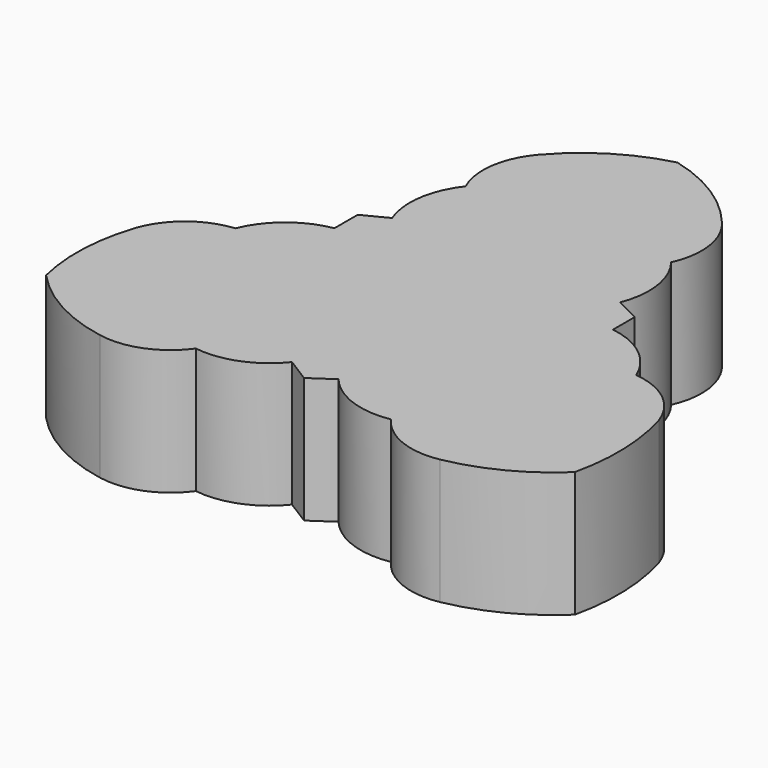
from build123d import *

# Parameters (mm, degrees)
F1_DEPTH = 11.1125


# Not quite as in the source:
# - a length typed as a fraction of an inch, garbled in the dataset ("3 / 203.2 mm" for 3/8 in), is restored


with BuildPart() as f1:
    # F0 (on Top) → F1 (new body)
    with BuildSketch(Plane.XY):
        with BuildLine():
            ThreePointArc((0, 27.0671695471), (-4.5048536548, 25.1556778504), (-8.2258973271, 21.977417171))
            ThreePointArc((-8.2258973271, 21.977417171), (-9.7181261566, 18.698842434), (-9.2097157612, 15.1327075437))
            ThreePointArc((-9.2097157612, 15.1327075437), (-10.6205392688, 11.8246856933), (-10.2093555033, 8.2519613206))
            Line((-10.2093555033, 8.2519613206), (-12.369341217, 7.1464567445))
            Line((-12.369341217, 7.1464567445), (-12.369341217, 4.6386048198))
            Line((-12.369341217, 4.6386048198), (-12.369341217, 4.5682978211))
            ThreePointArc((-12.369341217, 4.5682978211), (-15.5930977879, 3.1185654947), (-17.7027139134, 0.2823972963))
            ThreePointArc((-17.7027139134, 0.2823972963), (-21.0452825194, -1.0603738309), (-23.1384971151, -3.9919692741))
            ThreePointArc((-23.1384971151, -3.9919692741), (-23.9954710425, -8.6613028545), (-23.5336683691, -13.3861117065))
            ThreePointArc((-23.5336683691, -13.3861117065), (-19.6562098094, -16.4130421994), (-15.0192606046, -18.054899429))
            ThreePointArc((-15.0192606046, -18.054899429), (-11.4338171794, -17.7079201351), (-8.5996589687, -15.484556372))
            ThreePointArc((-8.5996589687, -15.484556372), (-5.0294162563, -15.0523544446), (-2.1409380715, -12.9098966718))
            Line((-2.1409380715, -12.9098966718), (0, -14.2561570176))
            Line((0, -14.2561570176), (1.9696742658, -12.9098966718))
            ThreePointArc((1.9696742658, -12.9098966718), (4.9392756736, -15.0084468105), (8.560301624, -15.3410370587))
            ThreePointArc((8.560301624, -15.3410370587), (11.3944598347, -17.5644008218), (14.9799032599, -17.9113801157))
            ThreePointArc((14.9799032599, -17.9113801157), (19.5156578324, -16.3470620723), (23.423301056, -13.563092798))
            ThreePointArc((23.423301056, -13.563092798), (23.8861103651, -8.6849198531), (23.0991397704, -3.8484499608))
            ThreePointArc((23.0991397704, -3.8484499608), (21.0059251747, -0.9168545176), (17.6633565687, 0.4259166096))
            ThreePointArc((17.6633565687, 0.4259166096), (15.4847616458, 3.3168082822), (12.1560195839, 4.739132713))
            Line((12.1560195839, 4.739132713), (12.1560195839, 7.1464567445))
            Line((12.1560195839, 7.1464567445), (9.9960338703, 8.2519613206))
            ThreePointArc((9.9960338703, 8.2519613206), (10.4072176357, 11.8246856933), (8.9963941282, 15.1327075437))
            ThreePointArc((8.9963941282, 15.1327075437), (9.5048045235, 18.698842434), (8.012575694, 21.977417171))
            ThreePointArc((8.012575694, 21.977417171), (4.4155385291, 25.1665589), (0, 27.0671695471))
        make_face()
    extrude(amount=F1_DEPTH)


solid = f1.part
